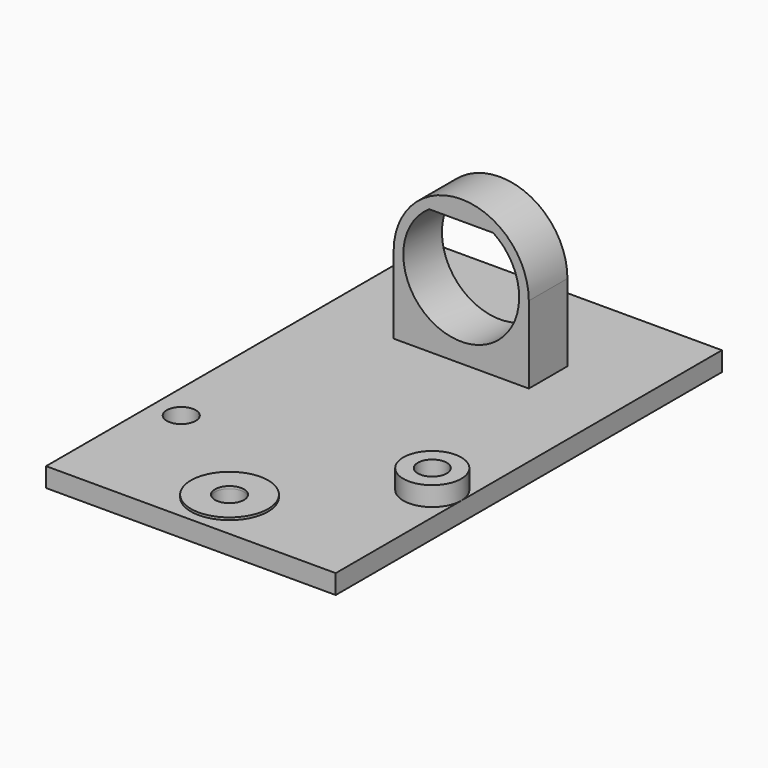
from build123d import *

# Parameters (mm, degrees)
F1_DEPTH = 5
F2_DEPTH = 15
F3_DEPTH = 35
F4_R     = 3
F4_R_2   = 1.5
F5_DEPTH = 2
F4_R_3   = 4
F6_DEPTH = 0.25
F7_DEPTH = 25


# Not quite as in the source:
# - a feature names something its author has since deleted; it is built from what else it names


with BuildPart() as f1:
    # F0 (on Front) → F1 (new body)
    with BuildSketch(Plane.XZ):
        with BuildLine():
            Line((7, 2), (7, 10))
            ThreePointArc((7, 10), (0, 17), (-7, 10))
            Line((-7, 10), (-7, 2))
            Line((-7, 2), (7, 2))
        make_face()
        with BuildLine():
            ThreePointArc((3.3166247904, 15), (0, 4), (-3.3166247904, 15))
            Line((-3.3166247904, 15), (3.3166247904, 15))
        make_face(mode=Mode.SUBTRACT)
    extrude(amount=-F1_DEPTH)

    # F0 (on Front) → F2 (join)
    with BuildSketch(Plane.XZ):
        Polygon((15, 2), (7, 2), (-7, 2), (-15, 2), (-15, 0), (15, 0), align=None)
    extrude(amount=-F2_DEPTH)

    # F0 (on Front) → F3 (join)
    with BuildSketch(Plane.XZ):
        Polygon((15, 2), (7, 2), (-7, 2), (-15, 2), (-15, 0), (15, 0), align=None)
    extrude(amount=F3_DEPTH)

    # F4 (on face) → F5 (join)
    with BuildSketch(Plane.XY.offset(2)):
        with Locations((12, -18.75)):
            Circle(F4_R)
        with Locations((12, -18.75)):
            Circle(F4_R_2, mode=Mode.SUBTRACT)
    extrude(amount=F5_DEPTH)

    # F4 (on face) → F6 (join)
    with BuildSketch(Plane.XY.offset(2)):
        with Locations((0, -30)):
            Circle(F4_R_3)
        with Locations((0, -30)):
            Circle(F4_R_2, mode=Mode.SUBTRACT)
    extrude(amount=F6_DEPTH)

    # F4 (on face) → F7 (cut)
    with BuildSketch(Plane.XY.offset(2)):
        with Locations((-12, -21.25)):
            Circle(F4_R_2)
        with Locations((0, -30)):
            Circle(F4_R_2)
        with Locations((12, -18.75)):
            Circle(F4_R_2)
    extrude(amount=-F7_DEPTH, mode=Mode.SUBTRACT)


solid = f1.part
